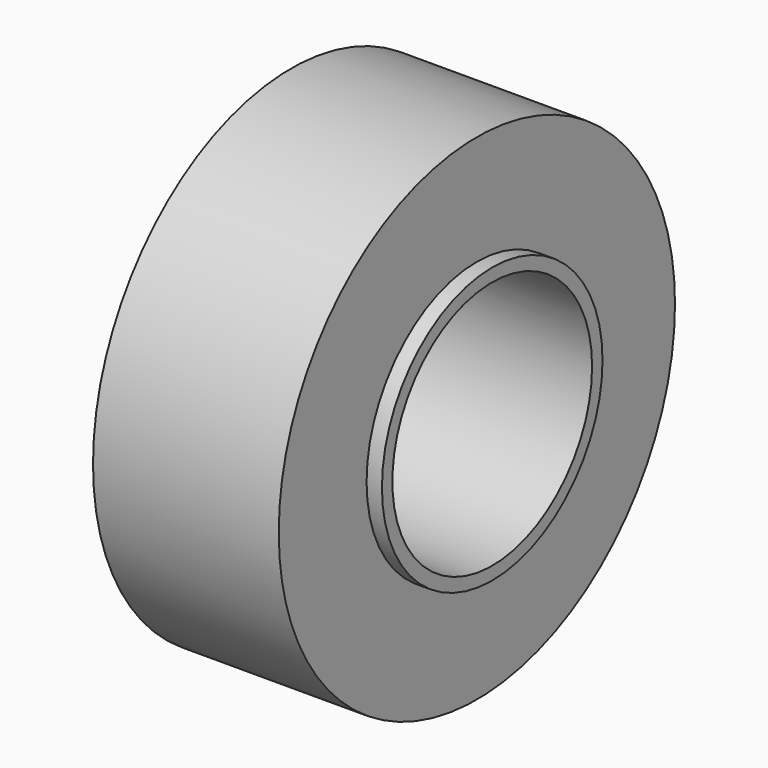
from build123d import *

# Parameters (mm, degrees)
F0_R     = 6.35
F0_R_2   = 3.2004
F1_DEPTH = 2.38125
F2_R     = 3.535
F2_R_2   = 3.2004
F3_DEPTH = 2.775


# Not quite as in the source:
# - a length typed as a fraction of an inch, garbled in the dataset ("3 / 203.2 mm" for 3/8 in), is restored


with BuildPart() as f1:
    # F0 (on Right) → F1 (new body, symmetric)
    with BuildSketch(Plane.YZ):
        Circle(F0_R)
        Circle(F0_R_2, mode=Mode.SUBTRACT)
    extrude(amount=F1_DEPTH, both=True)

    # F2 (on Right) → F3 (join, symmetric)
    with BuildSketch(Plane.YZ):
        Circle(F2_R)
        Circle(F2_R_2, mode=Mode.SUBTRACT)
    extrude(amount=F3_DEPTH, both=True)


solid = f1.part
